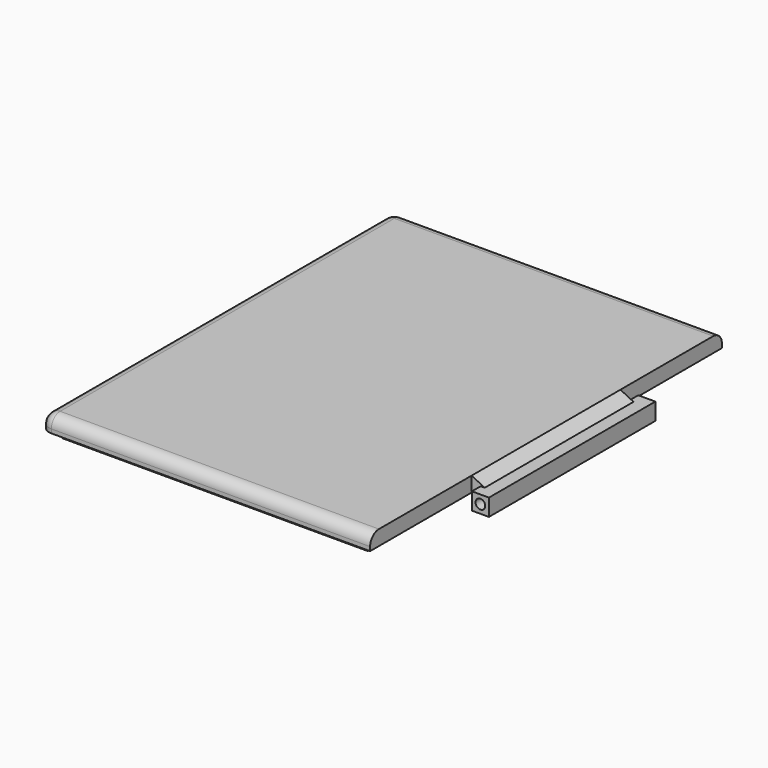
from build123d import *

# Parameters (mm, degrees)
F1_DEPTH     = 50.8
F2_DEPTH     = 48.006
F3_R         = 2.54
F4_T1_DEPTH  = 7.2669304909
F4_S5_W      = 2.54
F4_S5_H      = 2.54
F4_T6_DEPTH  = 2.54
F4_S11_W     = 2.54
F4_S11_H     = 2.54
F4_T12_DEPTH = 2.54
F0_R         = 1.1176
F5_DEPTH     = 24.0284
F6_DEPTH     = 21.4884


# Not quite as in the source:
# - a fillet or chamfer that OpenCascade refuses, or shapes differently, is made with other operations: its cross-section is extruded or revolved along the edge and cut away or added
# - ends of sketch curves that miss each other by under 0.0002 mm in the source are joined


with BuildPart() as f1:
    # F0 (on Front) → F1 (new body, symmetric)
    with BuildSketch(Plane.XZ):
        Polygon((35.306, -0.5352410823), (38.1, -0.5352410823), (38.1, -0.2915388458), (38.1, 2.9216894086), (-38.1, 2.9216894086), (-38.1, -0.5352410823), (-35.306, -0.5352410823), align=None)
    extrude(amount=F1_DEPTH, both=True)

    # F3
    f3_edges = [f1.edges().sort_by_distance(p)[0] for p in [
        (0, 50.8, 2.921689),
        (-38.1, 0, 2.921689),
        (0, -50.8, 2.921689),
    ]]
    fillet(f3_edges, radius=F3_R)

    # F4: fillet of radius 2.54 on 4 edges, made by hand

    # F4_s2 → F4_t1 (cut)
    with BuildSketch(Plane.XY.offset(-6.8852410823)):
        with BuildLine():
            ThreePointArc((-38.1, 48.26), (-37.3560512242, 50.0560512242), (-35.56, 50.8))
            Line((-35.56, 50.8), (-38.1, 50.8))
            Line((-38.1, 50.8), (-38.1, 48.26))
        make_face()
        with BuildLine():
            ThreePointArc((-38.1, -48.26), (-37.3560512242, -50.0560512242), (-35.56, -50.8))
            Line((-35.56, -50.8), (-38.1, -50.8))
            Line((-38.1, -50.8), (-38.1, -48.26))
        make_face()
    extrude(amount=F4_T1_DEPTH, mode=Mode.SUBTRACT)


with BuildPart() as f2:
    # F0 (on Front) → F2 (new body, symmetric)
    with BuildSketch(Plane.XZ):
        Polygon((35.306, -2.5619280059), (35.306, -0.5352806766), (-35.306, -0.5352410823), (-35.306, -2.5619280059), align=None)
    extrude(amount=F2_DEPTH, both=True)


with BuildPart() as f4_tool4:
    # F4_s5 → F4_t6 (new body)
    with BuildSketch(Plane.YZ.offset(-35.56)):
        with Locations((49.53, 1.6516894086)):
            Rectangle(F4_S5_W, F4_S5_H)
    extrude(amount=-F4_T6_DEPTH)

    # F4_s7 → F4_t8 (revolve, cut)
    with BuildSketch(Plane(origin=(-35.56, 48.26, 0.3816894086), x_dir=(0, -0.7071067812, -0.7071067812), z_dir=(0, 0.7071067812, -0.7071067812))):
        with BuildLine():
            ThreePointArc((0, -2.54), (2.54, 0), (0, 2.54))
            Line((0, 2.54), (0, -2.54))
        make_face()
    revolve(axis=Axis((-35.56, 48.26, 0.3816894086), (-1, 0, 0)), mode=Mode.SUBTRACT)


with BuildPart() as f1_1:
    add(f1.part)

    # F4_t3: cut F4_tool4
    add(f4_tool4.part, mode=Mode.SUBTRACT)


with BuildPart() as f4_tool10:
    # F4_s11 → F4_t12 (new body)
    with BuildSketch(Plane.YZ.offset(-35.56)):
        with Locations((-49.53, 1.6516894086)):
            Rectangle(F4_S11_W, F4_S11_H)
    extrude(amount=-F4_T12_DEPTH)

    # F4_s13 → F4_t14 (revolve, cut)
    with BuildSketch(Plane(origin=(-35.56, -48.26, 0.3816894086), x_dir=(0, 0.7071067812, -0.7071067812), z_dir=(0, 0.7071067812, 0.7071067812))):
        with BuildLine():
            ThreePointArc((0, -2.54), (2.54, 0), (0, 2.54))
            Line((0, 2.54), (0, -2.54))
        make_face()
    revolve(axis=Axis((-35.56, -48.26, 0.3816894086), (-1, 0, 0)), mode=Mode.SUBTRACT)


with BuildPart() as f1_2:
    add(f1_1.part)

    # F4_t9: cut F4_tool10
    add(f4_tool10.part, mode=Mode.SUBTRACT)


with BuildPart() as f5:
    # F0 (on Front) → F5 (new body, symmetric)
    with BuildSketch(Plane.XZ):
        with BuildLine():
            ThreePointArc((42.156539749, 0.9252589177), (40.7684698267, -0.0810141116), (41.2931384536, -1.7132047715))
            ThreePointArc((41.2931384536, -1.7132047715), (42.8168664325, -1.8379417083), (43.617039749, -0.5352410823))
            ThreePointArc((43.617039749, -0.5352410823), (43.1892692029, 0.4974883716), (42.156539749, 0.9252589177))
        make_face()
        with Locations((42.156539749, -0.5352410823)):
            Circle(F0_R, mode=Mode.SUBTRACT)
        with BuildLine():
            Line((40.1855779506, 1.4325042982), (40.1855779506, -1.2200908491))
            Line((40.1855779506, -1.2200908491), (41.2931384536, -1.7132047715))
            ThreePointArc((41.2931384536, -1.7132047715), (40.7684698267, -0.0810141116), (42.156539749, 0.9252589177))
            Line((42.156539749, 0.9252589177), (41.1258697318, 1.4325042982))
            Line((41.1258697318, 1.4325042982), (40.1855779506, 1.4325042982))
        make_face()
        with BuildLine():
            Line((41.2931384536, -1.7132047715), (40.1855779506, -1.2200908491))
            Line((40.1855779506, -1.2200908491), (40.1855779506, -2.5029864628))
            Line((40.1855779506, -2.5029864628), (44.1275015473, -2.5029864628))
            Line((44.1275015473, -2.5029864628), (44.1275015473, 1.4325042982))
            Line((44.1275015473, 1.4325042982), (41.1258697318, 1.4325042982))
            Line((41.1258697318, 1.4325042982), (42.156539749, 0.9252589177))
            ThreePointArc((42.156539749, 0.9252589177), (43.1892692029, 0.4974883716), (43.617039749, -0.5352410823))
            ThreePointArc((43.617039749, -0.5352410823), (42.8168664325, -1.8379417083), (41.2931384536, -1.7132047715))
        make_face()
    extrude(amount=F5_DEPTH, both=True)


with BuildPart() as f6:
    # F0 (on Front) → F6 (new body, symmetric)
    with BuildSketch(Plane.XZ):
        with BuildLine():
            Line((40.1855779506, 1.4325042982), (40.1855779506, -1.2200908491))
            Line((40.1855779506, -1.2200908491), (41.2931384536, -1.7132047715))
            ThreePointArc((41.2931384536, -1.7132047715), (40.7684698267, -0.0810141116), (42.156539749, 0.9252589177))
            Line((42.156539749, 0.9252589177), (41.1258697318, 1.4325042982))
            Line((41.1258697318, 1.4325042982), (40.1855779506, 1.4325042982))
        make_face()
        Polygon((38.1, 2.9216894086), (38.1, -0.2915388458), (40.1855779506, -1.2200908491), (40.1855779506, 1.4325042982), (41.1258697318, 1.4325042982), align=None)
    extrude(amount=F6_DEPTH, both=True)


solid = Compound([f2.part, f1_2.part, f5.part, f6.part])
